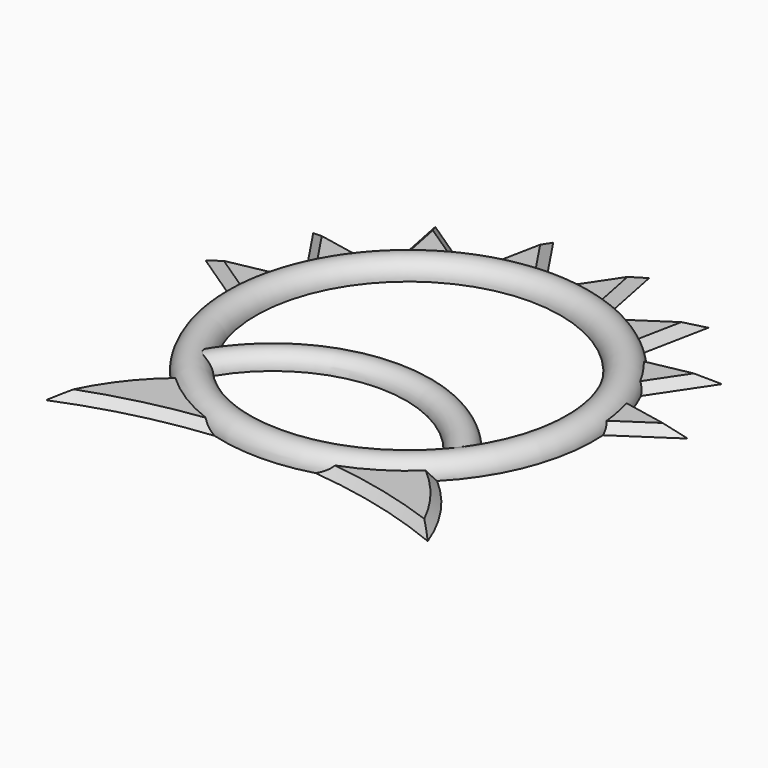
from build123d import *

# Parameters (mm, degrees)
F3_DEPTH      = 2
F4_SIZE       = 1.99999
F6_ANGLE_BACK = 65
F6_ANGLE      = 130


# Not quite as in the source:
# - a fillet or chamfer is up to 0.001 mm smaller than in the source, because OpenCascade refuses the exact size


with BuildPart() as f1:
    # F0 (on Right) → F1 (revolve)
    with BuildSketch(Plane.YZ):
        with BuildLine():
            Line((-44, 0), (-36, 0))
            ThreePointArc((-36, 0), (-40, 4), (-44, 0))
        make_face()
    revolve(axis=Axis((0, 0, -2.6855529286), (0, 0, -1)))

    # F2 (on Top) → F3 (join)
    with BuildSketch(Plane.XY):
        Polygon((-40, 0), (-36.9551813005, 15.3073372946), (-56.9551813005, 11.329089947), align=None)
        Polygon((-36.9551813005, 15.3073372946), (-28.2842712475, 28.2842712475), (-48.2842712475, 32.2625185951), align=None)
        Polygon((-28.2842712475, 28.2842712475), (-15.3073372946, 36.9551813005), (-32.2625185951, 48.2842712475), align=None)
        Polygon((-15.3073372946, 36.9551813005), (0, 40), (-11.329089947, 56.9551813005), align=None)
        Polygon((11.329089947, 56.9551813005), (0, 40), (15.3073372946, 36.9551813005), align=None)
        Polygon((32.2625185951, 48.2842712475), (15.3073372946, 36.9551813005), (28.2842712475, 28.2842712475), align=None)
        Polygon((48.2842712475, 32.2625185951), (28.2842712475, 28.2842712475), (36.9551813005, 15.3073372946), align=None)
        Polygon((56.9551813005, 11.329089947), (36.9551813005, 15.3073372946), (40, 0), align=None)
        with BuildLine():
            ThreePointArc((45.08495815, -50.6352676217), (38.3490901499, -38.208624723), (28.2842712475, -28.2842712475))
            Line((28.2842712475, -28.2842712475), (15.3073372946, -36.9551813005))
            Line((15.3073372946, -36.9551813005), (0, -40))
            Line((0, -40), (-15.3073372946, -36.9551813005))
            Line((-15.3073372946, -36.9551813005), (-28.2842712475, -28.2842712475))
            ThreePointArc((-28.2842712475, -28.2842712475), (-38.3490901499, -38.208624723), (-45.08495815, -50.6352676217))
            ThreePointArc((-45.08495815, -50.6352676217), (0, -41.7413833361), (45.08495815, -50.6352676217))
        make_face()
    extrude(amount=F3_DEPTH)

    # F4 (size 2 in the source; OpenCascade refuses exactly that, so slightly less here)
    f4_edges = [f1.edges().sort_by_distance(p)[0] for p in [
        (-50.179856, 6.801962, 2),
        (-48.96314, 12.918806, 2),
        (-40.29223, 30.672803, 2),
        (-43.757144, 25.487193, 2),
        (-25.487193, 43.757144, 2),
        (-30.672803, 40.29223, 2),
        (-6.801962, 50.179856, 2),
        (-12.918806, 48.96314, 2),
        (12.918806, 48.96314, 2),
        (6.801962, 50.179856, 2),
        (30.672803, 40.29223, 2),
        (25.487193, 43.757144, 2),
        (43.757144, 25.487193, 2),
        (40.29223, 30.672803, 2),
        (50.179856, 6.801962, 2),
        (48.96314, 12.918806, 2),
        (-39.37124, -39.621186, 2),
        (-28.06685, -45.10677, 2),
        (28.06685, -45.10677, 2),
        (39.37124, -39.621186, 2),
    ]]
    chamfer(f4_edges, length=F4_SIZE)

    # F5 (on Right) → F6 (revolve)
    with BuildSketch(Plane.YZ, mode=Mode.PRIVATE) as f6_sk:
        with BuildLine():
            Line((-8.5, 0), (-1.5, 0))
            ThreePointArc((-1.5, 0), (-5, 3.5), (-8.5, 0))
        make_face()
    revolve(f6_sk.sketch.rotate(Axis((0, -40, 2.6011376176), (0, 0, 1)), -F6_ANGLE_BACK), axis=Axis((0, -40, 2.6011376176), (0, 0, 1)), revolution_arc=F6_ANGLE)


solid = f1.part
